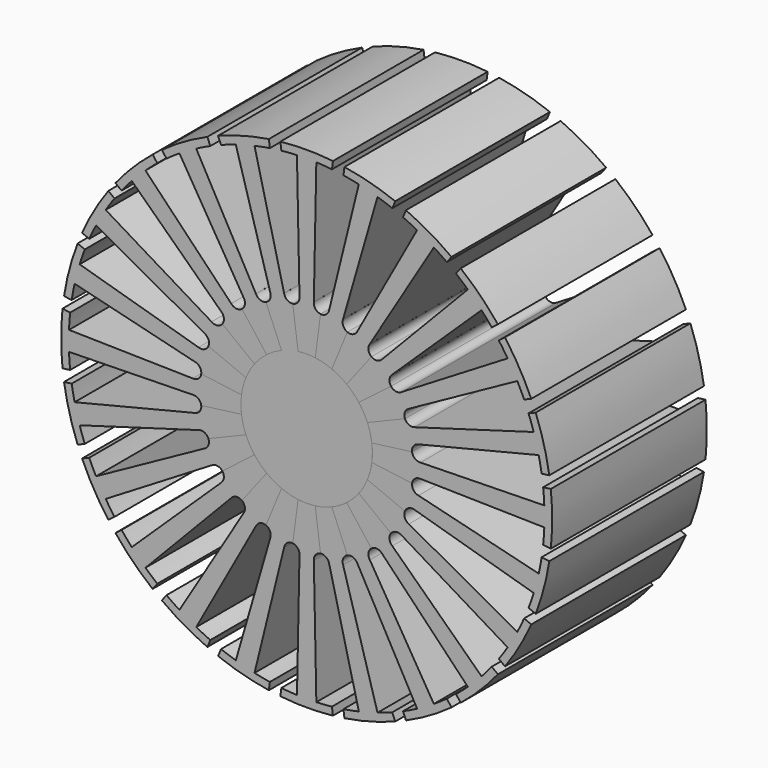
from build123d import *

# Parameters (mm, degrees)
F1_DEPTH = 50
F2_COUNT = 24


with BuildPart() as f1:
    # F0 (on Front) → F1 (new body)
    with BuildSketch(Plane.XZ):
        with BuildLine():
            ThreePointArc((-2.2189452677, 16.8545626434), (-11.2088788567, -12.7812767271), (17, 0))
            ThreePointArc((17, 0), (12.7812767271, 11.2088788567), (2.2189452677, 16.8545626434))
            Line((2.2189452677, 16.8545626434), (0, 0))
            Line((0, 0), (-2.2189452677, 16.8545626434))
        make_face()
        with BuildLine():
            Line((0, 0), (2.2189452677, 16.8545626434))
            ThreePointArc((2.2189452677, 16.8545626434), (0, 17), (-2.2189452677, 16.8545626434))
            Line((-2.2189452677, 16.8545626434), (0, 0))
        make_face()
        with BuildLine():
            ThreePointArc((-2.2189452677, 16.8545626434), (0, 17), (2.2189452677, 16.8545626434))
            Line((2.2189452677, 16.8545626434), (3.5894702861, 27.2647336878))
            ThreePointArc((3.5894702861, 27.2647336878), (2.2846829276, 28.0033782982), (1.8599233063, 29.4413091641))
            Line((1.8599233063, 29.4413091641), (1.8540318311, 29.4416807599))
            Line((1.8540318311, 29.4416807599), (2.5, 61.4491659829))
            ThreePointArc((2.5, 61.4491659829), (4.5213528869, 61.3335745581), (6.5378055, 61.1515093783))
            Line((6.5378055, 61.1515093783), (6.7989331193, 63.1349705665))
            ThreePointArc((6.7989331193, 63.1349705665), (0, 63.5), (-6.7989331193, 63.1349705665))
            Line((-6.7989331193, 63.1349705665), (-6.5378055, 61.1515093783))
            ThreePointArc((-6.5378055, 61.1515093783), (-4.5245926751, 61.3333356432), (-2.5064917867, 61.4489015274))
            Line((-2.5064917867, 61.4489015274), (-1.8599233063, 29.4413091641))
            ThreePointArc((-1.8599233063, 29.4413091641), (-2.2846829276, 28.0033782982), (-3.5894702861, 27.2647336878))
            Line((-3.5894702861, 27.2647336878), (-2.2189452677, 16.8545626434))
        make_face()
    extrude(amount=F1_DEPTH)


with BuildPart() as f2_1:
    # F2: instance of F1
    add(f1.part.rotate(Axis((0, 0, 0), (0, 1, 0)), 1 * 360 / F2_COUNT))


with BuildPart() as f2_2:
    # F2: instance of F1
    add(f1.part.rotate(Axis((0, 0, 0), (0, 1, 0)), 2 * 360 / F2_COUNT))


with BuildPart() as f2_3:
    # F2: instance of F1
    add(f1.part.rotate(Axis((0, 0, 0), (0, 1, 0)), 3 * 360 / F2_COUNT))


with BuildPart() as f2_4:
    # F2: instance of F1
    add(f1.part.rotate(Axis((0, 0, 0), (0, 1, 0)), 4 * 360 / F2_COUNT))


with BuildPart() as f2_5:
    # F2: instance of F1
    add(f1.part.rotate(Axis((0, 0, 0), (0, 1, 0)), 5 * 360 / F2_COUNT))


with BuildPart() as f2_6:
    # F2: instance of F1
    add(f1.part.rotate(Axis((0, 0, 0), (0, 1, 0)), 6 * 360 / F2_COUNT))


with BuildPart() as f2_7:
    # F2: instance of F1
    add(f1.part.rotate(Axis((0, 0, 0), (0, 1, 0)), 7 * 360 / F2_COUNT))


with BuildPart() as f2_8:
    # F2: instance of F1
    add(f1.part.rotate(Axis((0, 0, 0), (0, 1, 0)), 8 * 360 / F2_COUNT))


with BuildPart() as f2_9:
    # F2: instance of F1
    add(f1.part.rotate(Axis((0, 0, 0), (0, 1, 0)), 9 * 360 / F2_COUNT))


with BuildPart() as f2_10:
    # F2: instance of F1
    add(f1.part.rotate(Axis((0, 0, 0), (0, 1, 0)), 10 * 360 / F2_COUNT))


with BuildPart() as f2_11:
    # F2: instance of F1
    add(f1.part.rotate(Axis((0, 0, 0), (0, 1, 0)), 11 * 360 / F2_COUNT))


with BuildPart() as f2_12:
    # F2: instance of F1
    add(f1.part.rotate(Axis((0, 0, 0), (0, 1, 0)), 12 * 360 / F2_COUNT))


with BuildPart() as f2_13:
    # F2: instance of F1
    add(f1.part.rotate(Axis((0, 0, 0), (0, 1, 0)), 13 * 360 / F2_COUNT))


with BuildPart() as f2_14:
    # F2: instance of F1
    add(f1.part.rotate(Axis((0, 0, 0), (0, 1, 0)), 14 * 360 / F2_COUNT))


with BuildPart() as f2_15:
    # F2: instance of F1
    add(f1.part.rotate(Axis((0, 0, 0), (0, 1, 0)), 15 * 360 / F2_COUNT))


with BuildPart() as f2_16:
    # F2: instance of F1
    add(f1.part.rotate(Axis((0, 0, 0), (0, 1, 0)), 16 * 360 / F2_COUNT))


with BuildPart() as f2_17:
    # F2: instance of F1
    add(f1.part.rotate(Axis((0, 0, 0), (0, 1, 0)), 17 * 360 / F2_COUNT))


with BuildPart() as f2_18:
    # F2: instance of F1
    add(f1.part.rotate(Axis((0, 0, 0), (0, 1, 0)), 18 * 360 / F2_COUNT))


with BuildPart() as f2_19:
    # F2: instance of F1
    add(f1.part.rotate(Axis((0, 0, 0), (0, 1, 0)), 19 * 360 / F2_COUNT))


with BuildPart() as f2_20:
    # F2: instance of F1
    add(f1.part.rotate(Axis((0, 0, 0), (0, 1, 0)), 20 * 360 / F2_COUNT))


with BuildPart() as f2_21:
    # F2: instance of F1
    add(f1.part.rotate(Axis((0, 0, 0), (0, 1, 0)), 21 * 360 / F2_COUNT))


with BuildPart() as f2_22:
    # F2: instance of F1
    add(f1.part.rotate(Axis((0, 0, 0), (0, 1, 0)), 22 * 360 / F2_COUNT))


with BuildPart() as f2_23:
    # F2: instance of F1
    add(f1.part.rotate(Axis((0, 0, 0), (0, 1, 0)), 23 * 360 / F2_COUNT))


solid = Compound([f1.part, f2_1.part, f2_2.part, f2_3.part, f2_4.part, f2_5.part, f2_6.part, f2_7.part, f2_8.part, f2_9.part, f2_10.part, f2_11.part, f2_12.part, f2_13.part, f2_14.part, f2_15.part, f2_16.part, f2_17.part, f2_18.part, f2_19.part, f2_20.part, f2_21.part, f2_22.part, f2_23.part])
